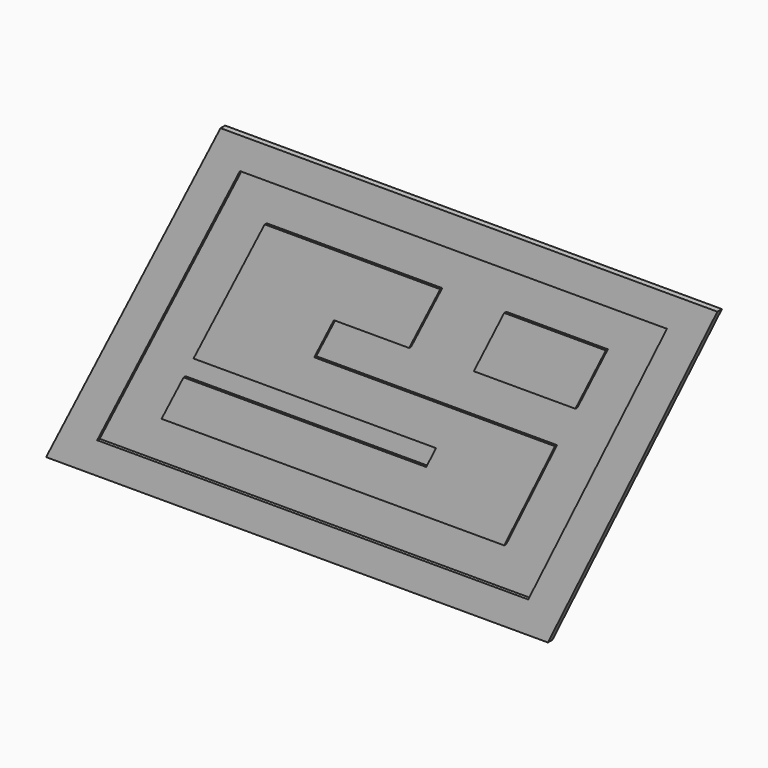
from build123d import *

# Parameters (mm, degrees)
F1_DEPTH = 0.4064
F3_DEPTH = 0.2032
F5_DEPTH = 0.4572
F6_SCALE = 4.5


# Not quite as in the source:
# - a feature names something its author has since deleted; it is built from what else it names


with BuildPart() as f1:
    # F0 (on Front) → F1 (new body)
    with BuildSketch(Plane.XZ):
        Polygon((1.7399819335, 32.9988971353), (-12.4273560941, 32.9988971353), (-18.1648561832, 21.6064513681), (1.4037427613, 21.6064513681), (0.6089702947, 20.0053038526), (-18.9712312321, 20.0053038526), (-20.7453668118, 16.4825599641), (6.9015445188, 16.4825599641), (11.0007077456, 24.8590362167), (-8.4278472578, 24.8590362167), (-6.8397070281, 28.0124656121), (-0.7713007088, 28.0124656121), align=None)
    extrude(amount=F1_DEPTH)


with BuildPart() as f1b:
    # F0 (on Front) → F1, piece 2 (new body)
    with BuildSketch(Plane.XZ):
        Polygon((15.0998709723, 32.9988971353), (6.9015445188, 32.9988971353), (4.449058262, 28.0581217034), (12.6473847156, 28.0581217034), align=None)
    extrude(amount=F1_DEPTH)


with BuildPart() as f3:
    # F2 (on Front) → F3 (new body)
    with BuildSketch(Plane.XZ):
        Polygon((-14.3832698171, 36.1738971353), (-25.8992879083, 13.3075599641), (8.8825950149, 13.3075599641), (20.0726044695, 36.1738971353), align=None)
    extrude(amount=F3_DEPTH)

    # F4 (on Front) → F5 (join)
    with BuildSketch(Plane.XZ):
        Polygon((-15.9480007955, 38.7138971353), (-30.0224247855, 10.7675599641), (10.4674354118, 10.7675599641), (24.1434244793, 38.7138971353), align=None)
        Polygon((-25.8992879083, 13.3075599641), (-14.3832698171, 36.1738971353), (20.0726044695, 36.1738971353), (8.8825950149, 13.3075599641), align=None, mode=Mode.SUBTRACT)
    extrude(amount=F5_DEPTH)


with BuildPart() as f3_1:
    # F6: moved
    add(f3.part.scale(F6_SCALE).moved(Location((23.9389745984, 0, -98.0436296425))))


with BuildPart() as f1b_1:
    # F6: moved
    add(f1b.part.scale(F6_SCALE).moved(Location((23.9389745984, 0, -98.0436296425))))


with BuildPart() as f1_1:
    # F6: moved
    add(f1.part.scale(F6_SCALE).moved(Location((23.9389745984, 0, -98.0436296425))))


solid = Compound([f3_1.part, f1b_1.part, f1_1.part])
